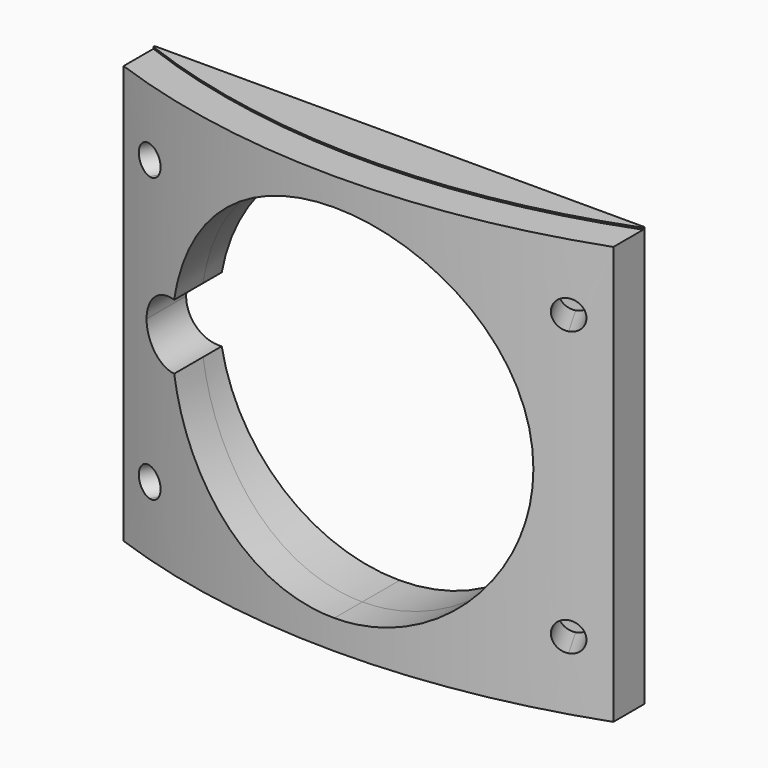
from build123d import *

# Parameters (mm, degrees)
F0_R           = 78.74
F0_R_2         = 74.93
F1_DEPTH       = 38.1
F2_R           = 1.5875
F3_DEPTH       = 177.8
F7_DEPTH       = 25.4
F8_W           = 170.1503526419
F8_H           = 177.0643368363
F9_DEPTH       = 76.2
F12_END_RADIUS = 74.93
F12_REACH      = 113.8647376176
F13_DEPTH      = 69.85
F15_DEPTH      = 8.8910001


with BuildPart() as f1:
    # F0 (on Top) → F1 (new body, symmetric)
    with BuildSketch(Plane.XY):
        Circle(F0_R)
        Circle(F0_R_2, mode=Mode.SUBTRACT)
    extrude(amount=F1_DEPTH, both=True)

    # F2 (on Front) → F3 (intersect)
    with BuildSketch(Plane.XZ):
        with BuildLine():
            ThreePointArc((-19.685, 15.4305), (-13.9193969877, 29.3498969877), (0, 35.1155))
            Line((0, 35.1155), (0, 38.2905))
            Line((0, 38.2905), (-26.6664084047, 38.2905))
            Line((-26.6664084047, 38.2905), (-26.6664084047, 15.4305))
            Line((-26.6664084047, 15.4305), (-19.685, 15.4305))
        make_face()
        with Locations((-23.8125, 30.861)):
            Circle(F2_R, mode=Mode.SUBTRACT)
        with BuildLine():
            Line((0, -7.4295), (0, -4.2545))
            ThreePointArc((0, -4.2545), (-13.9193969877, 1.5111030123), (-19.685, 15.4305))
            Line((-19.685, 15.4305), (-26.6664084047, 15.4305))
            Line((-26.6664084047, 15.4305), (-26.6664084047, -7.4295))
            Line((-26.6664084047, -7.4295), (0, -7.4295))
        make_face()
        with Locations((-23.8125, 0)):
            Circle(F2_R, mode=Mode.SUBTRACT)
        with BuildLine():
            Line((26.6664084047, 15.4305), (19.685, 15.4305))
            ThreePointArc((19.685, 15.4305), (13.9193969877, 1.5111030123), (0, -4.2545))
            Line((0, -4.2545), (0, -7.4295))
            Line((0, -7.4295), (26.6664084047, -7.4295))
            Line((26.6664084047, -7.4295), (26.6664084047, 15.4305))
        make_face()
        with Locations((23.8125, 0)):
            Circle(F2_R, mode=Mode.SUBTRACT)
        with BuildLine():
            ThreePointArc((0, 35.1155), (13.9193969877, 29.3498969877), (19.685, 15.4305))
            Line((19.685, 15.4305), (26.6664084047, 15.4305))
            Line((26.6664084047, 15.4305), (26.6664084047, 38.2905))
            Line((26.6664084047, 38.2905), (0, 38.2905))
            Line((0, 38.2905), (0, 35.1155))
        make_face()
        with Locations((23.8125, 30.861)):
            Circle(F2_R, mode=Mode.SUBTRACT)
        with Locations((-23.8125, 30.861)):
            Circle(F2_R)
        with Locations((23.8125, 30.861)):
            Circle(F2_R)
        with Locations((-23.8125, 0)):
            Circle(F2_R)
        with Locations((23.8125, 0)):
            Circle(F2_R)
    extrude(amount=F3_DEPTH, mode=Mode.INTERSECT)

    # F6 (on face) → F7 (cut)
    with BuildSketch(Plane(origin=(38.7472337077, -67.1121774345, 0), x_dir=(-0.8660254038, -0.5, 0), z_dir=(-0.5, 0.8660254038, 0))):
        with BuildLine():
            ThreePointArc((19.5060294768, 0), (19.041061492, 1.1225320151), (17.9185294768, 1.5875))
            Line((17.9185294768, 1.5875), (17.9185294768, -1.5875))
            ThreePointArc((17.9185294768, -1.5875), (19.041061492, -1.1225320151), (19.5060294768, 0))
        make_face()
        with BuildLine():
            Line((17.9185294768, -1.5875), (17.9185294768, 1.5875))
            ThreePointArc((17.9185294768, 1.5875), (16.3310294768, 0), (17.9185294768, -1.5875))
        make_face()
        with BuildLine():
            ThreePointArc((19.5060294768, 30.861), (19.041061492, 31.9835320151), (17.9185294768, 32.4485))
            Line((17.9185294768, 32.4485), (17.9185294768, 29.2735))
            ThreePointArc((17.9185294768, 29.2735), (19.041061492, 29.7384679849), (19.5060294768, 30.861))
        make_face()
        with BuildLine():
            Line((17.9185294768, 29.2735), (17.9185294768, 32.4485))
            ThreePointArc((17.9185294768, 32.4485), (16.3310294768, 30.861), (17.9185294768, 29.2735))
        make_face()
    extrude(amount=F7_DEPTH, mode=Mode.SUBTRACT)

    # F8 (on Right) → F9 (cut)
    with BuildSketch(Plane.YZ):
        with Locations((-62.6385295764, 18.013317138)):
            Rectangle(F8_W, F8_H)
    extrude(amount=-F9_DEPTH, mode=Mode.SUBTRACT)

    # F10: F1 across plane


with BuildPart() as f1_1:
    add(f1.part)
    add(f1.part.mirror(Plane.YZ))

    f12_end = (Plane(origin=(0, 0, 15.33525), x_dir=(-1, 0, 0), z_dir=(0, 0, -1)) * Cylinder(F12_END_RADIUS, 369.0558714917, mode=Mode.PRIVATE)).faces().sort_by_distance((0, -74.93, -6.7265497667))[0]
    # F2 (on Front) → F12 (join, up to the whole of a round face its end follows)
    with BuildSketch(Plane.XZ):
        with BuildLine():
            ThreePointArc((0, 35.1155), (13.9193969877, 29.3498969877), (19.685, 15.4305))
            Line((19.685, 15.4305), (26.6664084047, 15.4305))
            Line((26.6664084047, 15.4305), (26.6664084047, 38.2905))
            Line((26.6664084047, 38.2905), (0, 38.2905))
            Line((0, 38.2905), (0, 35.1155))
        make_face()
        with Locations((23.8125, 30.861)):
            Circle(F2_R, mode=Mode.SUBTRACT)
        with BuildLine():
            ThreePointArc((-19.685, 15.4305), (-13.9193969877, 29.3498969877), (0, 35.1155))
            Line((0, 35.1155), (0, 38.2905))
            Line((0, 38.2905), (-26.6664084047, 38.2905))
            Line((-26.6664084047, 38.2905), (-26.6664084047, 15.4305))
            Line((-26.6664084047, 15.4305), (-19.685, 15.4305))
        make_face()
        with Locations((-23.8125, 30.861)):
            Circle(F2_R, mode=Mode.SUBTRACT)
        with BuildLine():
            Line((0, -7.4295), (0, -4.2545))
            ThreePointArc((0, -4.2545), (-13.9193969877, 1.5111030123), (-19.685, 15.4305))
            Line((-19.685, 15.4305), (-26.6664084047, 15.4305))
            Line((-26.6664084047, 15.4305), (-26.6664084047, -7.4295))
            Line((-26.6664084047, -7.4295), (0, -7.4295))
        make_face()
        with Locations((-23.8125, 0)):
            Circle(F2_R, mode=Mode.SUBTRACT)
        with BuildLine():
            Line((26.6664084047, 15.4305), (19.685, 15.4305))
            ThreePointArc((19.685, 15.4305), (13.9193969877, 1.5111030123), (0, -4.2545))
            Line((0, -4.2545), (0, -7.4295))
            Line((0, -7.4295), (26.6664084047, -7.4295))
            Line((26.6664084047, -7.4295), (26.6664084047, 15.4305))
        make_face()
        with Locations((23.8125, 0)):
            Circle(F2_R, mode=Mode.SUBTRACT)
        with Locations((-23.8125, 0)):
            Circle(F2_R)
        with Locations((-23.8125, 30.861)):
            Circle(F2_R)
        with Locations((23.8125, 30.861)):
            Circle(F2_R)
        with Locations((23.8125, 0)):
            Circle(F2_R)
    f12_long = extrude(amount=F12_REACH, mode=Mode.PRIVATE)
    add(split(f12_long, bisect_by=f12_end, keep=Keep.BOTTOM, mode=Mode.PRIVATE))

    # F2 (on Front) → F13 (cut)
    with BuildSketch(Plane.XZ):
        with BuildLine():
            Line((26.6664084047, 15.4305), (19.685, 15.4305))
            ThreePointArc((19.685, 15.4305), (13.9193969877, 1.5111030123), (0, -4.2545))
            Line((0, -4.2545), (0, -7.4295))
            Line((0, -7.4295), (26.6664084047, -7.4295))
            Line((26.6664084047, -7.4295), (26.6664084047, 15.4305))
        make_face()
        with Locations((23.8125, 0)):
            Circle(F2_R, mode=Mode.SUBTRACT)
        with BuildLine():
            ThreePointArc((-19.685, 15.4305), (-13.9193969877, 29.3498969877), (0, 35.1155))
            Line((0, 35.1155), (0, 38.2905))
            Line((0, 38.2905), (-26.6664084047, 38.2905))
            Line((-26.6664084047, 38.2905), (-26.6664084047, 15.4305))
            Line((-26.6664084047, 15.4305), (-19.685, 15.4305))
        make_face()
        with Locations((-23.8125, 30.861)):
            Circle(F2_R, mode=Mode.SUBTRACT)
        with BuildLine():
            Line((0, -7.4295), (0, -4.2545))
            ThreePointArc((0, -4.2545), (-13.9193969877, 1.5111030123), (-19.685, 15.4305))
            Line((-19.685, 15.4305), (-26.6664084047, 15.4305))
            Line((-26.6664084047, 15.4305), (-26.6664084047, -7.4295))
            Line((-26.6664084047, -7.4295), (0, -7.4295))
        make_face()
        with Locations((-23.8125, 0)):
            Circle(F2_R, mode=Mode.SUBTRACT)
        with BuildLine():
            ThreePointArc((0, 35.1155), (13.9193969877, 29.3498969877), (19.685, 15.4305))
            Line((19.685, 15.4305), (26.6664084047, 15.4305))
            Line((26.6664084047, 15.4305), (26.6664084047, 38.2905))
            Line((26.6664084047, 38.2905), (0, 38.2905))
            Line((0, 38.2905), (0, 35.1155))
        make_face()
        with Locations((23.8125, 30.861)):
            Circle(F2_R, mode=Mode.SUBTRACT)
        with Locations((-23.8125, 0)):
            Circle(F2_R)
        with Locations((23.8125, 0)):
            Circle(F2_R)
        with Locations((23.8125, 30.861)):
            Circle(F2_R)
        with Locations((-23.8125, 30.861)):
            Circle(F2_R)
    extrude(amount=F13_DEPTH, mode=Mode.SUBTRACT)

    # F14 (on face) → F15 (cut, through all)
    with BuildSketch(Plane(origin=(0, -69.85, 0), x_dir=(-1, 0, 0), z_dir=(0, 1, 0))):
        with BuildLine():
            ThreePointArc((19.3638129032, 18.971965071), (19.6045387857, 17.2085), (19.685, 15.4305))
            ThreePointArc((19.685, 15.4305), (19.6045387857, 13.6525), (19.3638129032, 11.889034929))
            ThreePointArc((19.3638129032, 11.889034929), (22.0832279587, 12.8049260326), (23.241, 15.4305))
            ThreePointArc((23.241, 15.4305), (22.0832279587, 18.0560739674), (19.3638129032, 18.971965071))
        make_face()
        with BuildLine():
            ThreePointArc((19.3638129032, 11.889034929), (19.6045387857, 13.6525), (19.685, 15.4305))
            Line((19.685, 15.4305), (16.129, 15.4305))
            ThreePointArc((16.129, 15.4305), (17.0594260326, 13.0322720413), (19.3638129032, 11.889034929))
        make_face()
    extrude(amount=-F15_DEPTH, mode=Mode.SUBTRACT)


solid = f1_1.part
